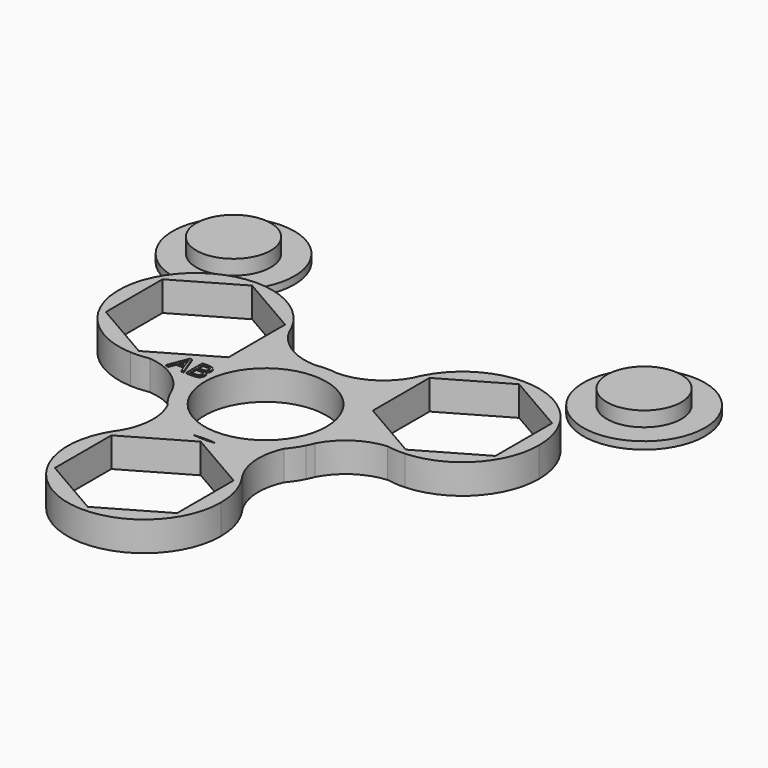
from build123d import *

# Parameters (mm, degrees)
F0_R         = 14.6025460528
F2_DEPTH     = 7.112
F1_R         = 8.9311105539
F3_DEPTH     = 5.334
F4_DEPTH     = 5.334
F1_R_2       = 14.6025460528
F5_DEPTH     = 1.778
F6_DEPTH     = 1.778
F7_TEXT_SIZE = 6.6793898845
F8_DEPTH     = 7.35


# Not quite as in the source:
# - Text() gives the source's letters only with a copy of the font that has no kerning and outlines rounded to 1/6400 em; it was checked with that copy


with BuildPart() as f2:
    # F0 (on Top) → F2 (new body)
    with BuildSketch(Plane.XY):
        with BuildLine():
            ThreePointArc((17.1713824713, -6.5694097025), (18.0791573253, -3.3402979239), (18.3851439977, 0))
            ThreePointArc((18.3851439977, 0), (13.9086511871, 12.023433036), (2.6590836535, 18.191833166))
            ThreePointArc((2.6590836535, 18.191833166), (1.3250047881, 18.2260794283), (0, 18.3851439977))
            ThreePointArc((0, 18.3851439977), (-1.3250047881, 18.2260794283), (-2.6590836535, 18.191833166))
            ThreePointArc((-2.6590836535, 18.191833166), (-15.8616403244, 9.2963372376), (-17.1713824713, -6.5694097025))
            ThreePointArc((-17.1713824713, -6.5694097025), (-16.7486562372, -7.4399783526), (-16.386077271, -8.3372652281))
            ThreePointArc((-16.386077271, -8.3372652281), (-15.0486597548, -10.043651276), (-13.9859762509, -11.9333980124))
            ThreePointArc((-13.9859762509, -11.9333980124), (-8.8982787147, -16.0883235836), (-2.6746988703, -18.1895438582))
            ThreePointArc((-2.6746988703, -18.1895438582), (0, -17.9939437187), (2.6746988703, -18.1895438582))
            ThreePointArc((2.6746988703, -18.1895438582), (8.8982787147, -16.0883235836), (13.9859762509, -11.9333980124))
            ThreePointArc((13.9859762509, -11.9333980124), (15.0486597548, -10.043651276), (16.386077271, -8.3372652281))
            ThreePointArc((16.386077271, -8.3372652281), (16.7486562372, -7.4399783526), (17.1713824713, -6.5694097025))
        make_face()
        Circle(F0_R, mode=Mode.SUBTRACT)
        with BuildLine():
            ThreePointArc((2.6590836535, 18.191833166), (13.9086511871, 12.023433036), (18.3851439977, 0))
            ThreePointArc((18.3851439977, 0), (18.0791573253, -3.3402979239), (17.1713824713, -6.5694097025))
            ThreePointArc((17.1713824713, -6.5694097025), (21.8928082303, -1.3547571237), (28.5351214621, 0.9613036801))
            ThreePointArc((28.5351214621, 0.9613036801), (15.934426476, 10.1076268428), (14.8697435247, 25.6414348674))
            ThreePointArc((14.8697435247, 25.6414348674), (9.7683930698, 20.2710088615), (2.6590836535, 18.191833166))
        make_face()
        with BuildLine():
            ThreePointArc((0, 18.3851439977), (1.3250047881, 18.2260794283), (2.6590836535, 18.191833166))
            ThreePointArc((2.6590836535, 18.191833166), (1.3330505386, 18.3367526044), (0, 18.3851439977))
        make_face()
        with BuildLine():
            ThreePointArc((16.386077271, -8.3372652281), (16.8019970354, -7.4636730526), (17.1713824713, -6.5694097025))
            ThreePointArc((17.1713824713, -6.5694097025), (16.7486562372, -7.4399783526), (16.386077271, -8.3372652281))
        make_face()
        with BuildLine():
            ThreePointArc((-2.6590836535, 18.191833166), (-1.3250047881, 18.2260794283), (0, 18.3851439977))
            ThreePointArc((0, 18.3851439977), (-1.3330505386, 18.3367526044), (-2.6590836535, 18.191833166))
        make_face()
        with BuildLine():
            ThreePointArc((15.7123341697, 27.5057426814), (15.3245849851, 26.5584272964), (14.8697435247, 25.6414348674))
            ThreePointArc((14.8697435247, 25.6414348674), (15.934426476, 10.1076268428), (28.5351214621, 0.9613036801))
            ThreePointArc((28.5351214621, 0.9613036801), (30.7513928105, 0.9785954322), (32.9434700761, 0.6515557465))
            ThreePointArc((32.9434700761, 0.6515557465), (45.3418328161, 6.3443750862), (50.4037347162, 19.01342161))
            ThreePointArc((50.4037347162, 19.01342161), (36.3901262098, 36.8712825475), (15.7123341697, 27.5057426814))
        make_face()
        Polygon((32.0185907185, 35.9980637528), (46.7277222884, 27.5057426814), (46.7277222884, 10.5211005386), (32.0185907185, 2.0287794672), (17.3094591486, 10.5211005386), (17.3094591486, 27.5057426814), align=None, mode=Mode.SUBTRACT)
        with BuildLine():
            ThreePointArc((15.7123341697, 27.5057426814), (15.2650865324, 26.5853181559), (14.8697435247, 25.6414348674))
            ThreePointArc((14.8697435247, 25.6414348674), (15.3245849851, 26.5584272964), (15.7123341697, 27.5057426814))
        make_face()
        with BuildLine():
            ThreePointArc((13.9859762509, -11.9333980124), (15.292104222, -10.2061289566), (16.386077271, -8.3372652281))
            ThreePointArc((16.386077271, -8.3372652281), (15.0486597548, -10.043651276), (13.9859762509, -11.9333980124))
        make_face()
        with BuildLine():
            ThreePointArc((32.9434700761, 0.6515557465), (30.7513928105, 0.9785954322), (28.5351214621, 0.9613036801))
            ThreePointArc((28.5351214621, 0.9613036801), (30.7299551947, 0.6734941755), (32.9434700761, 0.6515557465))
        make_face()
        with BuildLine():
            ThreePointArc((-17.1713824713, -6.5694097025), (-15.8616403244, 9.2963372376), (-2.6590836535, 18.191833166))
            ThreePointArc((-2.6590836535, 18.191833166), (-9.7683930698, 20.2710088615), (-14.8697435247, 25.6414348674))
            ThreePointArc((-14.8697435247, 25.6414348674), (-13.945163472, 22.3845857089), (-13.6334467208, 19.01342161))
            ThreePointArc((-13.6334467208, 19.01342161), (-17.8401281131, 7.3093745338), (-28.5351214621, 0.9613036801))
            ThreePointArc((-28.5351214621, 0.9613036801), (-21.8928082303, -1.3547571237), (-17.1713824713, -6.5694097025))
        make_face()
        with BuildLine():
            ThreePointArc((14.8616003089, -25.5556706924), (12.683854813, -18.8563752793), (13.9859762509, -11.9333980124))
            ThreePointArc((13.9859762509, -11.9333980124), (8.8982787147, -16.0883235836), (2.6746988703, -18.1895438582))
            ThreePointArc((2.6746988703, -18.1895438582), (9.5102788266, -20.6447902597), (14.8616003089, -25.5556706924))
        make_face()
        with BuildLine():
            ThreePointArc((-16.386077271, -8.3372652281), (-16.7486562372, -7.4399783526), (-17.1713824713, -6.5694097025))
            ThreePointArc((-17.1713824713, -6.5694097025), (-16.8019970354, -7.4636730526), (-16.386077271, -8.3372652281))
        make_face()
        with BuildLine():
            ThreePointArc((-15.7123341697, 27.5057426814), (-15.3245849851, 26.5584272964), (-14.8697435247, 25.6414348674))
            ThreePointArc((-14.8697435247, 25.6414348674), (-15.2650865324, 26.5853181559), (-15.7123341697, 27.5057426814))
        make_face()
        with BuildLine():
            ThreePointArc((-13.6334467208, 19.01342161), (-13.945163472, 22.3845857089), (-14.8697435247, 25.6414348674))
            ThreePointArc((-14.8697435247, 25.6414348674), (-15.3245849851, 26.5584272964), (-15.7123341697, 27.5057426814))
            ThreePointArc((-15.7123341697, 27.5057426814), (-47.4922305637, 28.9421672386), (-32.9434700761, 0.6515557465))
            ThreePointArc((-32.9434700761, 0.6515557465), (-30.7513928105, 0.9785954322), (-28.5351214621, 0.9613036801))
            ThreePointArc((-28.5351214621, 0.9613036801), (-17.8401281131, 7.3093745338), (-13.6334467208, 19.01342161))
        make_face()
        Polygon((-32.0185907185, 35.9980637528), (-17.3094591486, 27.5057426814), (-17.3094591486, 10.5211005386), (-32.0185907185, 2.0287794672), (-46.7277222884, 10.5211005386), (-46.7277222884, 27.5057426814), align=None, mode=Mode.SUBTRACT)
        with BuildLine():
            ThreePointArc((14.8616003089, -25.5556706924), (9.5102788266, -20.6447902597), (2.6746988703, -18.1895438582))
            ThreePointArc((2.6746988703, -18.1895438582), (0, -18.3851439977), (-2.6746988703, -18.1895438582))
            ThreePointArc((-2.6746988703, -18.1895438582), (-9.5102788266, -20.6447902597), (-14.8616003089, -25.5556706924))
            ThreePointArc((-14.8616003089, -25.5556706924), (-15.1487702969, -25.9913791295), (-15.4517217151, -26.416266035))
            ThreePointArc((-15.4517217151, -26.416266035), (-5.1928504249, -54.0156356858), (18.3851439977, -36.3790877163))
            ThreePointArc((18.3851439977, -36.3790877163), (17.6365479695, -31.1862372914), (15.4517217151, -26.416266035))
            ThreePointArc((15.4517217151, -26.416266035), (15.1487702969, -25.9913791295), (14.8616003089, -25.5556706924))
        make_face()
        Polygon((0, -19.4485264994), (14.6622961142, -27.9138071078), (14.6622961142, -44.8443683248), (0, -53.3096489333), (-14.6622961142, -44.8443683248), (-14.6622961142, -27.9138071078), align=None, mode=Mode.SUBTRACT)
        with BuildLine():
            ThreePointArc((15.4517217151, -26.416266035), (15.1627678581, -25.98178082), (14.8616003089, -25.5556706924))
            ThreePointArc((14.8616003089, -25.5556706924), (15.1487702969, -25.9913791295), (15.4517217151, -26.416266035))
        make_face()
        with BuildLine():
            ThreePointArc((-13.9859762509, -11.9333980124), (-15.0486597548, -10.043651276), (-16.386077271, -8.3372652281))
            ThreePointArc((-16.386077271, -8.3372652281), (-15.292104222, -10.2061289566), (-13.9859762509, -11.9333980124))
        make_face()
        with BuildLine():
            ThreePointArc((-32.9434700761, 0.6515557465), (-30.7299551947, 0.6734941755), (-28.5351214621, 0.9613036801))
            ThreePointArc((-28.5351214621, 0.9613036801), (-30.7513928105, 0.9785954322), (-32.9434700761, 0.6515557465))
        make_face()
        with BuildLine():
            ThreePointArc((-14.8616003089, -25.5556706924), (-9.5102788266, -20.6447902597), (-2.6746988703, -18.1895438582))
            ThreePointArc((-2.6746988703, -18.1895438582), (-8.8982787147, -16.0883235836), (-13.9859762509, -11.9333980124))
            ThreePointArc((-13.9859762509, -11.9333980124), (-12.683854813, -18.8563752793), (-14.8616003089, -25.5556706924))
        make_face()
        with BuildLine():
            ThreePointArc((-15.4517217151, -26.416266035), (-15.1487702969, -25.9913791295), (-14.8616003089, -25.5556706924))
            ThreePointArc((-14.8616003089, -25.5556706924), (-15.1627678581, -25.98178082), (-15.4517217151, -26.416266035))
        make_face()
    extrude(amount=F2_DEPTH)

    # F7 (on Top) → F8 (join)
    with BuildSketch(Plane.XY):
        with Locations((-24.1960892454, 0.4508583806)):
            Text('AB', F7_TEXT_SIZE, font='Open Sans', text_align=(TextAlign.LEFT, TextAlign.BOTTOM))
    extrude(amount=F8_DEPTH)


with BuildPart() as f3:
    # F1 (on Top) → F3 (new body)
    with BuildSketch(Plane.XY):
        with Locations((-49.2382124066, 51.9467256963)):
            Circle(F1_R)
    extrude(amount=F3_DEPTH)

    # F1 (on Top) → F5 (join)
    with BuildSketch(Plane.XY):
        with Locations((-49.2382124066, 51.9467256963)):
            Circle(F1_R_2)
        with Locations((-49.2382124066, 51.9467256963)):
            Circle(F1_R, mode=Mode.SUBTRACT)
    extrude(amount=F5_DEPTH)


with BuildPart() as f4:
    # F1 (on Top) → F4 (new body)
    with BuildSketch(Plane.XY):
        with Locations((49.2382124066, 51.9467256963)):
            Circle(F1_R)
    extrude(amount=F4_DEPTH)

    # F1 (on Top) → F6 (join)
    with BuildSketch(Plane.XY):
        with Locations((49.2382124066, 51.9467256963)):
            Circle(F1_R_2)
        with Locations((49.2382124066, 51.9467256963)):
            Circle(F1_R, mode=Mode.SUBTRACT)
    extrude(amount=F6_DEPTH)


solid = Compound([f2.part, f3.part, f4.part])
